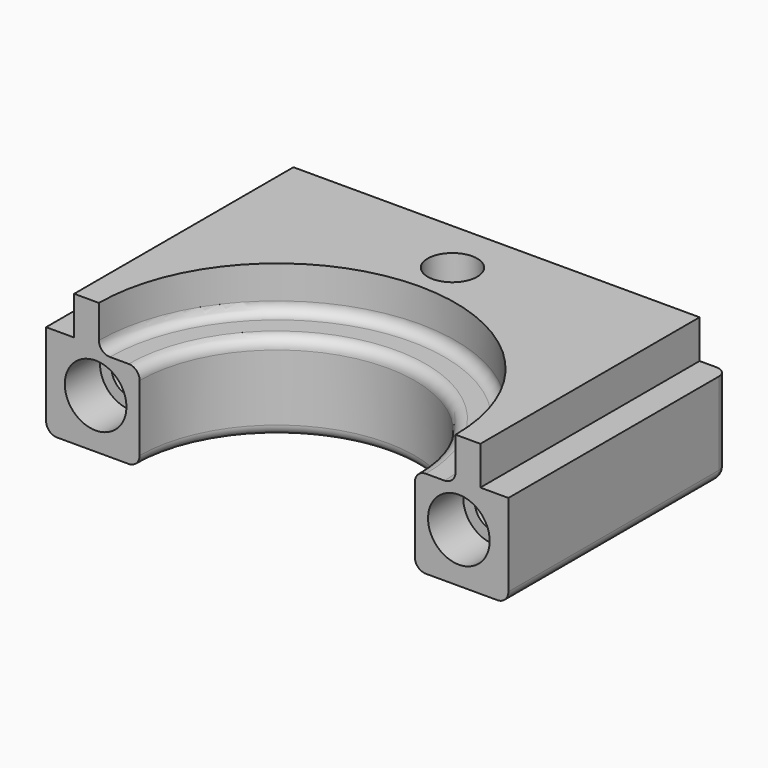
from build123d import *

# Parameters (mm, degrees)
F0_W      = 42
F0_H      = 24.9
F1_DEPTH  = 12
F3_DEPTH  = 4
F5_DEPTH  = 8
F7_D      = 4.5
F8_W      = 2.55
F8_H      = 3.5
F9_DEPTH  = 24.9
F12_D     = 3.5
F14_DEPTH = 3.5
F15_R     = 2.8
F15_R_2   = 1.75
F16_DEPTH = 4
F17_R     = 1.75
F18_DEPTH = 12
F19_R     = 1


# Not quite as in the source:
# - a pattern or mirror of a feature is missing from the dataset's text; its kind, count and spacing are read off the source's solid


with BuildPart() as f1:
    # F0 (on Top) → F1 (new body)
    with BuildSketch(Plane.XY):
        with Locations((0, 12.45)):
            Rectangle(F0_W, F0_H)
    extrude(amount=F1_DEPTH)

    # F2 (on face) → F3 (cut)
    with BuildSketch(Plane.XY.offset(12)):
        with BuildLine():
            Line((-16.2, 0), (16.2, 0))
            ThreePointArc((16.2, 0), (0, 16.2), (-16.2, 0))
        make_face()
    extrude(amount=-F3_DEPTH, mode=Mode.SUBTRACT)

    # F4 (on face) → F5 (cut, through all)
    with BuildSketch(Plane.XY.offset(8)):
        with BuildLine():
            Line((-12.5, 0), (12.5, 0))
            ThreePointArc((12.5, 0), (0, 12.5), (-12.5, 0))
        make_face()
    extrude(amount=-F5_DEPTH, mode=Mode.SUBTRACT)

    # F7 (through all)
    with Locations(Plane.XY.offset(12)):
        with Locations((0, 19.9)):
            Hole(F7_D / 2)

    # F8 (on face) → F9 (cut, through all)
    with BuildSketch(Plane.XZ):
        with Locations((-19.725, 10.25)):
            Rectangle(F8_W, F8_H)
    f9 = extrude(amount=-F9_DEPTH, mode=Mode.SUBTRACT)

    # F9_copies: F9 across plane
    add(f9.mirror(Plane(origin=(0, 0, 0), x_dir=(0, 0, 1), z_dir=(1, 0, 0))), mode=Mode.SUBTRACT)

    # F12 (through all)
    with Locations(Plane.XZ):
        with Locations((-16.5, 4.5), (16.5, 4.5)):
            Hole(F12_D / 2)

    # F13 (on face) → F14 (cut)
    with BuildSketch(Plane.XY):
        Polygon((-2.0005186827, 23.365), (-4.0010373655, 19.9), (-2.0005186827, 16.435), (2.0005186827, 16.435), (4.0010373655, 19.9), (2.0005186827, 23.365), align=None)
    extrude(amount=F14_DEPTH, mode=Mode.SUBTRACT)

    # F15 (on face) → F16 (cut)
    with BuildSketch(Plane.XZ):
        with Locations((16.5, 4.5)):
            Circle(F15_R)
        with Locations((16.5, 4.5)):
            Circle(F15_R_2, mode=Mode.SUBTRACT)
    f16 = extrude(amount=-F16_DEPTH, mode=Mode.SUBTRACT)

    # F16_copies: F16 across plane
    add(f16.mirror(Plane(origin=(0, 0, 0), x_dir=(0, 0, -1), z_dir=(-1, 0, 0))), mode=Mode.SUBTRACT)

    # F17 (on face) → F18 (cut)
    with BuildSketch(Plane(origin=(0, 24.9, 0), x_dir=(-1, 0, 0), z_dir=(0, 1, 0))):
        Polygon((-19.6927469886, 4.5), (-18.0963734943, 1.735), (-14.9036265057, 1.735), (-13.3072530114, 4.5), (-14.9036265057, 7.265), (-18.0963734943, 7.265), align=None)
        with Locations((-16.5, 4.5)):
            Circle(F17_R, mode=Mode.SUBTRACT)
    f18 = extrude(amount=-F18_DEPTH, mode=Mode.SUBTRACT)

    # F18_copies: F18 across plane
    add(f18.mirror(Plane(origin=(0, 0, 0), x_dir=(0, 0, -1), z_dir=(-1, 0, 0))), mode=Mode.SUBTRACT)

    # F19
    f19_edges = [f1.edges().sort_by_distance(p)[0] for p in [
        (21, 24.9, 4.25),
        (0, 24.9, 0),
        (-21, 24.9, 4.25),
        (-21, 12.45, 0),
        (21, 12.45, 0),
        (0, 12.5, 0),
        (0, 12.5, 8),
        (0, 16.2, 8),
    ]]
    fillet(f19_edges, radius=F19_R)


solid = f1.part
